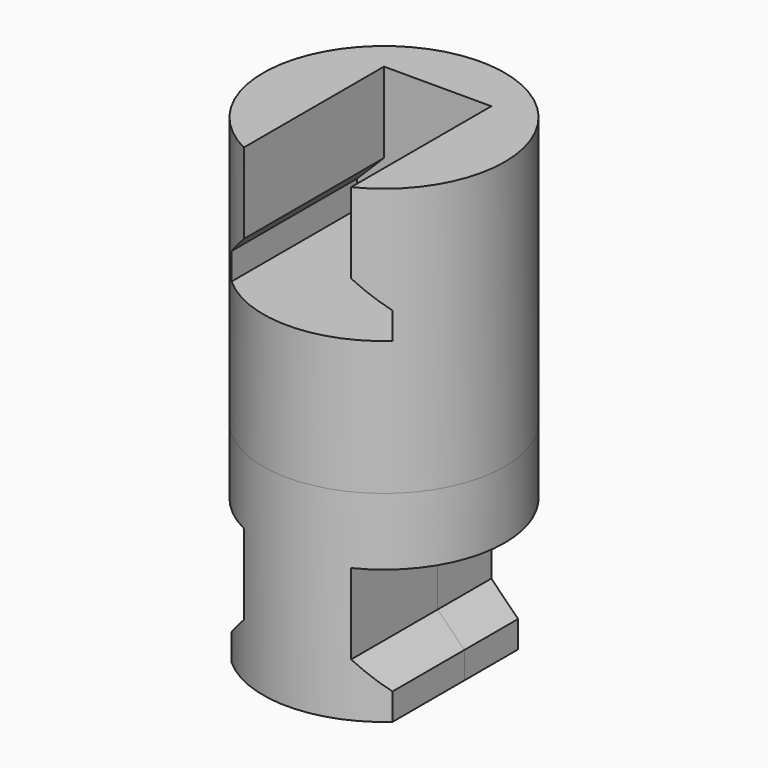
from build123d import *

# Parameters (mm, degrees)
F0_R          = 9
F1_DEPTH      = 20
F3_DEPTH      = 5
F3_DEPTH_BACK = 25
F4_DEPTH      = 15
F5_DEPTH      = 25
F5_DEPTH_BACK = 25
F6_W          = 13.7853547931
F6_H          = 8
F7_DEPTH      = 10
F8_SIZE2      = 1.99999
F8_SIZE       = 1.99999


# Not quite as in the source:
# - a fillet or chamfer is up to 0.001 mm smaller than in the source, because OpenCascade refuses the exact size


with BuildPart() as f1:
    # F0 (on Top) → F1 (new body)
    with BuildSketch(Plane.XY):
        Circle(F0_R)
    extrude(amount=F1_DEPTH)

    # F2 (on Front) → F3 (cut, two sides)
    with BuildSketch(Plane.XZ) as f3_sk:
        Polygon((0, 10), (0, 20), (-4, 20), (-4, 12), (-6, 12), (-6, 10), align=None)
        Polygon((4, 20), (0, 20), (0, 10), (6, 10), (6, 12), (4, 12), align=None)
        Polygon((-6, -15), (0, -15), (0, -5), (-4, -5), (-4, -13), (-6, -13), align=None)
        Polygon((0, -5), (0, -15), (6, -15), (6, -13), (4, -13), (4, -5), align=None)
        Polygon((6, -13), (6, -15), (9, -15), (9, -5), (4, -5), (4, -13), align=None)
        Polygon((-9, -15), (-6, -15), (-6, -13), (-4, -13), (-4, -5), (-9, -5), align=None)
    extrude(amount=-F3_DEPTH, mode=Mode.SUBTRACT)
    extrude(f3_sk.sketch, amount=F3_DEPTH_BACK, mode=Mode.SUBTRACT)

    # F4 (add): a face of the model
    f4_faces = [f1.faces().sort_by_distance(p)[0] for p in [
        (0, 0, 0),
    ]]
    extrude(f4_faces, amount=F4_DEPTH)

    # F2 (on Front) → F5 (cut, two sides)
    with BuildSketch(Plane.XZ) as f5_sk:
        Polygon((-9, -15), (-6, -15), (-6, -13), (-4, -13), (-4, -5), (-9, -5), align=None)
        Polygon((6, -13), (6, -15), (9, -15), (9, -5), (4, -5), (4, -13), align=None)
    extrude(amount=-F5_DEPTH, mode=Mode.SUBTRACT)
    extrude(f5_sk.sketch, amount=F5_DEPTH_BACK, mode=Mode.SUBTRACT)

    # F6 (on face) → F7 (cut)
    with BuildSketch(Plane(origin=(0, 0, -15), x_dir=(1, 0, 0), z_dir=(0, 0, -1))):
        with Locations((0, -9)):
            Rectangle(F6_W, F6_H)
    extrude(amount=-F7_DEPTH, mode=Mode.SUBTRACT)

    # F8 (size 2 and 2 in the source; OpenCascade refuses exactly that, so slightly less here)
    f8_edges = [f1.edges().sort_by_distance(p)[0] for p in [
        (4, -1.531129, 12),
        (-4, -1.531129, 12),
        (-4, -1.531129, -13),
        (4, -1.531129, -13),
    ]]
    chamfer(f8_edges, length=F8_SIZE, length2=F8_SIZE2)


solid = f1.part
